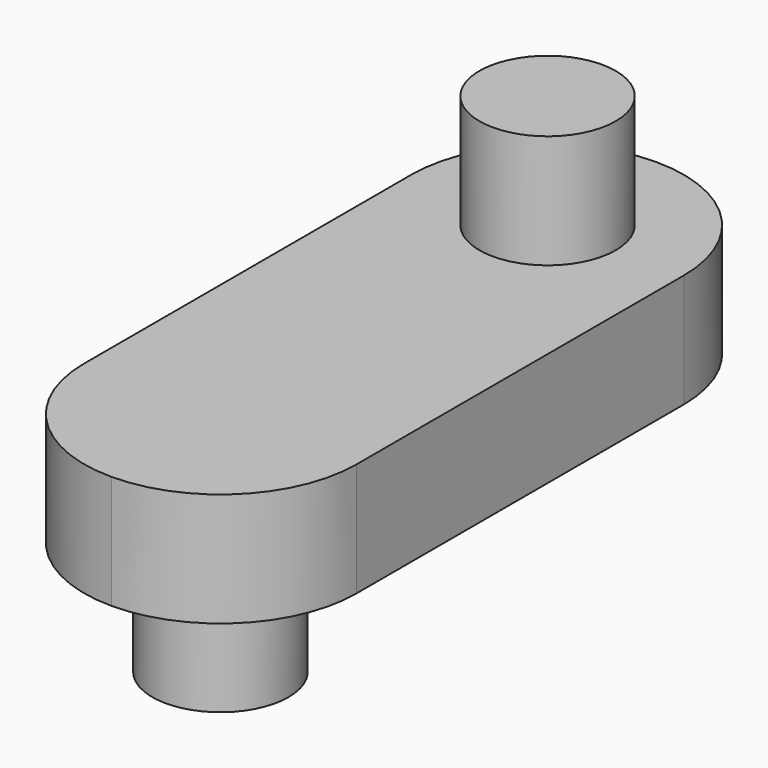
from build123d import *

# Parameters (mm, degrees)
F0_W     = 12
F0_H     = 30
F0_R     = 3
F1_DEPTH = 5
F2_DEPTH = 10
F3_DEPTH = 5
F4_R     = 5.99999


# Not quite as in the source:
# - a fillet or chamfer is up to 0.001 mm smaller than in the source, because OpenCascade refuses the exact size


with BuildPart() as f1:
    # F0 (on Top) → F1 (new body)
    with BuildSketch(Plane.XY):
        with Locations((0.0119865412, -0.4361811298)):
            Rectangle(F0_W, F0_H)
        with Locations((0.0119865412, -9.4361811298)):
            Circle(F0_R, mode=Mode.SUBTRACT)
        with Locations((0.0119865412, 8.5638188702)):
            Circle(F0_R, mode=Mode.SUBTRACT)
        with Locations((0.0119865412, 8.5638188702)):
            Circle(F0_R)
        with Locations((0.0119865412, -9.4361811298)):
            Circle(F0_R)
    extrude(amount=F1_DEPTH)

    # F0 (on Top) → F2 (join)
    with BuildSketch(Plane.XY):
        with Locations((0.0119865412, 8.5638188702)):
            Circle(F0_R)
    extrude(amount=F2_DEPTH)

    # F0 (on Top) → F3 (join)
    with BuildSketch(Plane.XY):
        with Locations((0.0119865412, -9.4361811298)):
            Circle(F0_R)
    extrude(amount=-F3_DEPTH)

    # F4 (radius 6 in the source; OpenCascade refuses exactly that, so slightly less here)
    f4_edges = [f1.edges().sort_by_distance(p)[0] for p in [
        (6.011987, 14.563819, 2.5),
        (-5.988013, 14.563819, 2.5),
        (6.011987, -15.436181, 2.5),
        (-5.988013, -15.436181, 2.5),
    ]]
    fillet(f4_edges, radius=F4_R)


solid = f1.part
